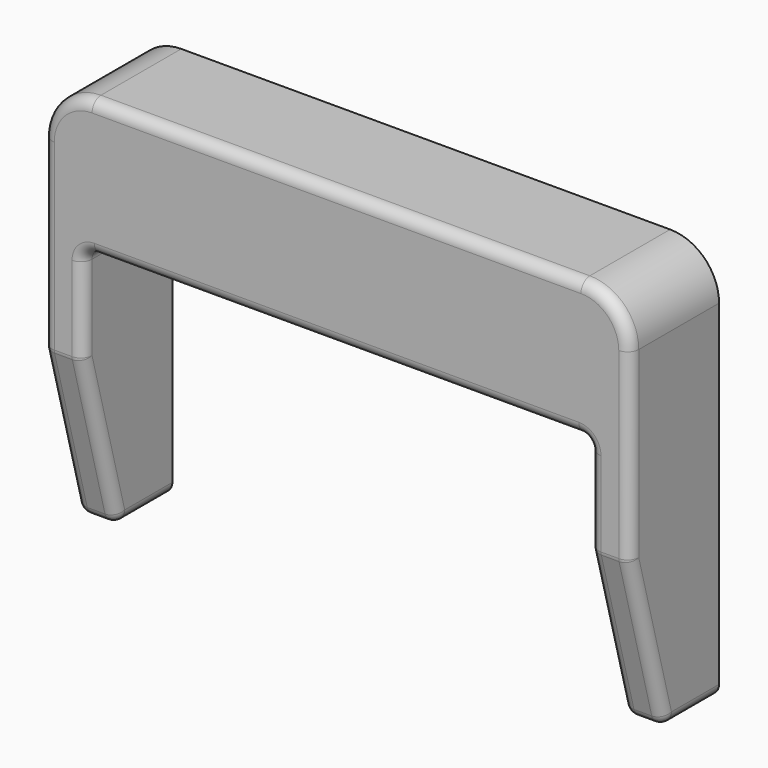
from build123d import *

# Parameters (mm, degrees)
F1_DEPTH    = 1.9558
F2_SIZE2    = 2.8438227154
F2_SIZE     = 0.762
F2_2_SIZE2  = 2.8438227154
F2_2_SIZE   = 0.762
F3_R        = 0.1950302499
F4_T1_DEPTH = 4.1020358569
F4_T4_ANGLE = 90
F4_T6_ANGLE = 90


# Not quite as in the source:
# - a fillet or chamfer that OpenCascade refuses, or shapes differently, is made with other operations: its cross-section is extruded or revolved along the edge and cut away or added


with BuildPart() as f1:
    # F0 (on Front) → F1 (new body)
    with BuildSketch(Plane.XZ):
        Polygon((-37.9921731242, 36.4987568722), (-48.2858929149, 36.4987568722), (-48.2858929149, 34.1091437473), (-48.2858929149, 29.5576006174), (-47.5840330195, 29.5576006174), (-47.5840330195, 34.1091437473), (-43.1390330195, 34.1091437473), (-38.6940330195, 34.1091437473), (-38.6940330195, 29.5576006174), (-37.9921731242, 29.5576006174), (-37.9921731242, 34.1091437473), align=None)
    extrude(amount=F1_DEPTH)

    # F2
    f2_edges = [f1.edges().sort_by_distance(p)[0] for p in [
        (-47.934963, -1.9558, 29.557601),
    ]]
    f2_side = f1.faces().sort_by_distance((-47.934963, -0.9779, 29.557601))[0]
    chamfer(f2_edges, length=F2_SIZE, length2=F2_SIZE2, reference=f2_side)

    # F2#2
    f2_2_edges = [f1.edges().sort_by_distance(p)[0] for p in [
        (-38.343103, -1.9558, 29.557601),
    ]]
    f2_2_side = f1.faces().sort_by_distance((-38.343103, -0.9779, 29.557601))[0]
    chamfer(f2_2_edges, length=F2_2_SIZE, length2=F2_2_SIZE2, reference=f2_2_side)

    # F3
    f3_edges = [f1.edges().sort_by_distance(p)[0] for p in [
        (-47.934963, -1.1938, 29.557601),
        (-38.343103, -1.1938, 29.557601),
        (-37.992173, -1.5748, 30.979512),
        (-38.694033, -1.5748, 30.979512),
        (-38.343103, -1.9558, 32.401423),
        (-43.139033, -1.9558, 34.109144),
        (-47.584033, -1.5748, 30.979512),
        (-48.285893, -1.5748, 30.979512),
        (-47.934963, -1.9558, 32.401423),
        (-47.584033, -1.9558, 33.255284),
        (-38.694033, -1.9558, 33.255284),
        (-37.992173, -1.9558, 34.45009),
        (-38.694033, -0.5969, 29.557601),
        (-37.992173, -0.5969, 29.557601),
        (-38.694033, -0.9779, 34.109144),
        (-47.584033, -0.9779, 34.109144),
        (-47.584033, -0.5969, 29.557601),
        (-48.285893, -0.5969, 29.557601),
        (-48.285893, -1.9558, 34.45009),
        (-43.139033, -1.9558, 36.498757),
    ]]
    fillet(f3_edges, radius=F3_R)

    # F4: fillet of radius 0.8584943428 on 2 edges, made by hand

    # F4_s2 → F4_t1 (cut)
    with BuildSketch(Plane.XZ.offset(-2.1462358569)):
        with BuildLine():
            ThreePointArc((-37.9921731242, 35.6402625294), (-38.2436202956, 36.2473097008), (-38.850667467, 36.4987568722))
            Line((-38.850667467, 36.4987568722), (-37.9921731242, 36.4987568722))
            Line((-37.9921731242, 36.4987568722), (-37.9921731242, 35.6402625294))
        make_face()
        with BuildLine():
            ThreePointArc((-47.4273985721, 36.4987568722), (-48.0344457435, 36.2473097008), (-48.2858929149, 35.6402625294))
            Line((-48.2858929149, 35.6402625294), (-48.2858929149, 36.4987568722))
            Line((-48.2858929149, 36.4987568722), (-47.4273985721, 36.4987568722))
        make_face()
    extrude(amount=F4_T1_DEPTH, mode=Mode.SUBTRACT)

    # F4_s3 → F4_t4 (revolve, cut)
    with BuildSketch(Plane.YZ.offset(-47.4273985721)):
        with BuildLine():
            ThreePointArc((-1.9558, 36.3037266223), (-1.8986769623, 36.4416338345), (-1.7607697501, 36.4987568722))
            Line((-1.7607697501, 36.4987568722), (-1.9558, 36.4987568722))
            Line((-1.9558, 36.4987568722), (-1.9558, 36.3037266223))
        make_face()
    revolve(axis=Axis((-47.4273985721, -1.9558, 35.6402625294), (0, -1, 0)), revolution_arc=F4_T4_ANGLE, mode=Mode.SUBTRACT)

    # F4_s5 → F4_t6 (revolve, cut)
    with BuildSketch(Plane.XY.offset(35.6402625294)):
        with BuildLine():
            ThreePointArc((-38.1872033741, -1.9558), (-38.0492961619, -1.8986769623), (-37.9921731242, -1.7607697501))
            Line((-37.9921731242, -1.7607697501), (-37.9921731242, -1.9558))
            Line((-37.9921731242, -1.9558), (-38.1872033741, -1.9558))
        make_face()
    revolve(axis=Axis((-38.850667467, -1.9558, 35.6402625294), (0, -1, 0)), revolution_arc=F4_T6_ANGLE, mode=Mode.SUBTRACT)


solid = f1.part
